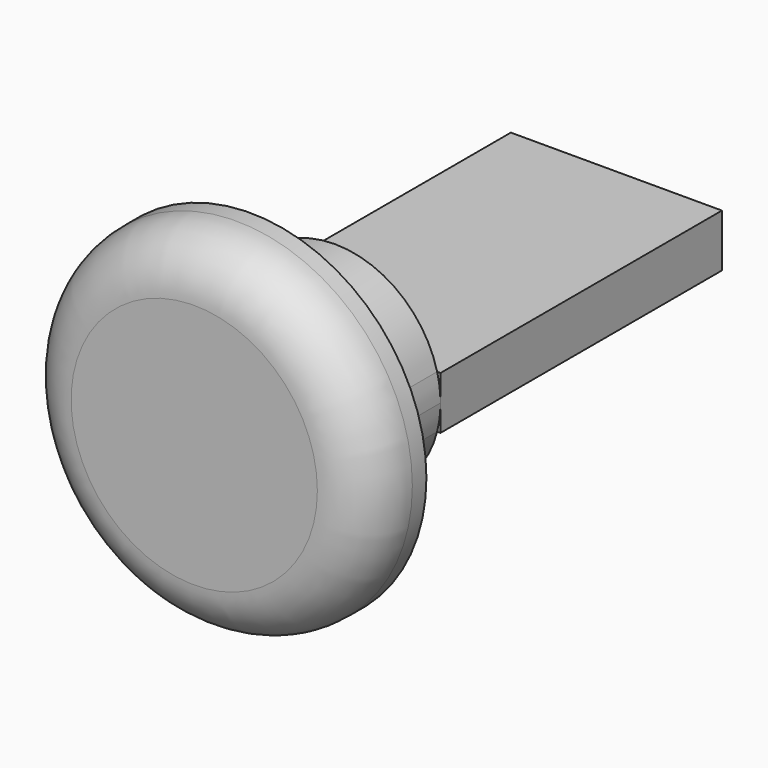
from build123d import *

# Parameters (mm, degrees)
F0_W     = 60
F0_H     = 15
F1_DEPTH = 100
F3_DEPTH = 30
F4_R     = 50
F4_R_2   = 30
F5_DEPTH = 20
F6_R     = 15
F8_DEPTH = 30


# Not quite as in the source:
# - a feature names something its author has since deleted; it is built from what else it names


with BuildPart() as f1:
    # F0 (on Front) → F1 (new body)
    with BuildSketch(Plane.XZ):
        Rectangle(F0_W, F0_H)
    extrude(amount=-F1_DEPTH)

    # F2 (on face) → F3 (join)
    with BuildSketch(Plane.XZ):
        with BuildLine():
            ThreePointArc((29.0473750966, -7.5), (29.760890888, -3.7801287745), (30, 0))
            ThreePointArc((30, 0), (29.760890888, 3.7801287745), (29.0473750966, 7.5))
            Line((29.0473750966, 7.5), (-29.0473750966, 7.5))
            ThreePointArc((-29.0473750966, 7.5), (-29.760890888, 3.7801287745), (-30, 0))
            ThreePointArc((-30, 0), (-29.760890888, -3.7801287745), (-29.0473750966, -7.5))
            Line((-29.0473750966, -7.5), (29.0473750966, -7.5))
        make_face()
        with BuildLine():
            Line((-29.0473750966, 7.5), (29.0473750966, 7.5))
            ThreePointArc((29.0473750966, 7.5), (0, 30), (-29.0473750966, 7.5))
        make_face()
        with BuildLine():
            ThreePointArc((-29.0473750966, -7.5), (0, -30), (29.0473750966, -7.5))
            Line((29.0473750966, -7.5), (-29.0473750966, -7.5))
        make_face()
    extrude(amount=F3_DEPTH)

    # F4 (on face) → F5 (join)
    with BuildSketch(Plane.XZ.offset(30)):
        Circle(F4_R)
        Circle(F4_R_2, mode=Mode.SUBTRACT)
        Circle(F4_R_2)
    extrude(amount=F5_DEPTH)

    # F6
    f6_edges = [f1.edges().sort_by_distance(p)[0] for p in [
        (-50, -50, 0),
    ]]
    fillet(f6_edges, radius=F6_R)

    # F7 (on face) → F8 (cut)
    with BuildSketch(Plane(origin=(0, 0, 0), x_dir=(-1, 0, 0), z_dir=(0, 1, 0))):
        with BuildLine():
            Line((5, -15), (-5, -15))
            Line((-5, -15), (-5, -29.5803989155))
            ThreePointArc((-5, -29.5803989155), (0, -30), (5, -29.5803989155))
            Line((5, -29.5803989155), (5, -15))
        make_face()
    extrude(amount=-F8_DEPTH, mode=Mode.SUBTRACT)


solid = f1.part
